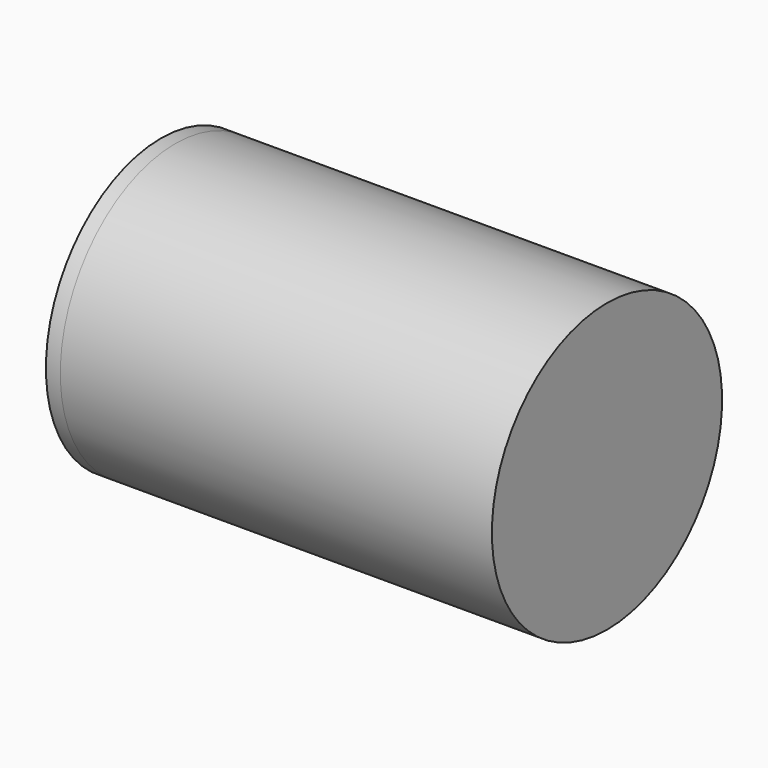
from build123d import *


# Not quite as in the source:
# - a feature names something its author has since deleted; it is built from what else it names


with BuildPart() as f1:
    # F0 (on Front) → F1 (revolve)
    with BuildSketch(Plane.XZ):
        Polygon((56, -2), (60, -2), (60, 2), (-60, 2), (-60, -2), align=None)
        Polygon((60, -38), (60, -2), (56, -2), (56, -9), (56, -11), (56, -38), align=None)
    revolve(axis=Axis((58, 0, -38), (-1, 0, 0)))


with BuildPart() as f2:
    # F0 (on Front) → F2 (revolve)
    with BuildSketch(Plane.XZ):
        Polygon((56, -11), (56, -9), (-60, -9), (-60, -10.997527279), (-60, -11), align=None)
        Polygon((-60, -9), (-60, -2), (-60, 2), (-64, 2), (-64, -10.997527279), (-60, -10.997527279), align=None)
    revolve(axis=Axis((58, 0, -38), (-1, 0, 0)))


solid = Compound([f1.part, f2.part])
